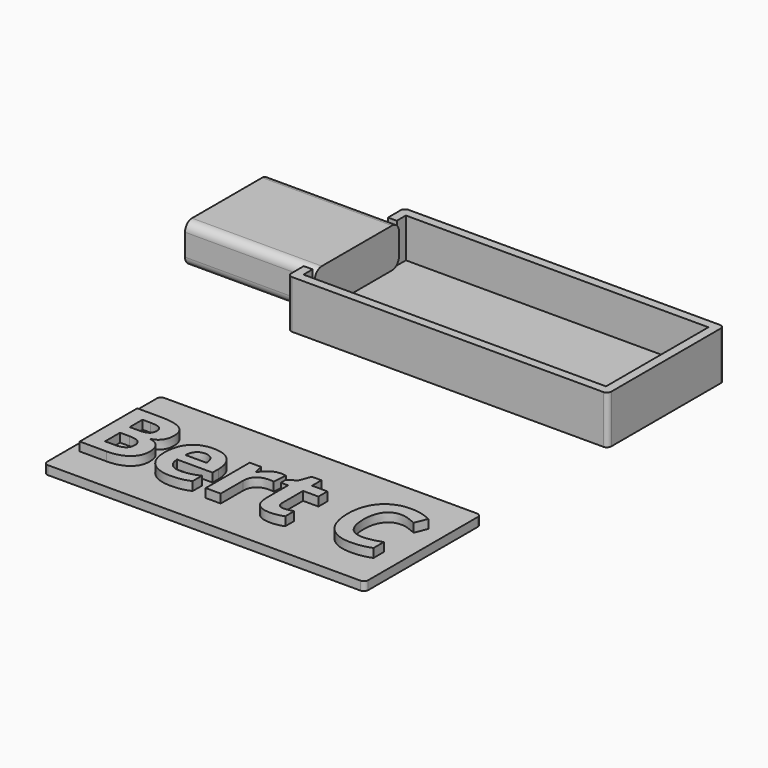
from build123d import *

# Parameters (mm, degrees)
F0_W         = 14.8
F0_H         = 6
F1_DEPTH     = 4.5
F2_R         = 1
F4_W         = 36.5
F4_H         = 16.6
F5_DEPTH     = 1
F6_DEPTH     = 4.5
F7_DEPTH     = 2
F8_R         = 0.5
F9_W         = 36.6
F9_H         = 16.6
F9_TEXT_SIZE = 11.4848814895
F10_DEPTH    = 1
F11_DEPTH    = 1
F12_R        = 0.5


# Not quite as in the source:
# - Text() gives the source's letters only with a copy of the font that has no kerning and outlines rounded to 1/6400 em; it was checked with that copy


with BuildPart() as f1:
    # F0 (on Top) → F1 (new body)
    with BuildSketch(Plane.XY):
        with Locations((-28.2312738687, -1.3390618086)):
            Rectangle(F0_W, F0_H)
        with Locations((-28.2312738687, -7.3390618086)):
            Rectangle(F0_W, F0_H)
    extrude(amount=F1_DEPTH)

    # F2
    f2_edges = [f1.edges().sort_by_distance(p)[0] for p in [
        (-28.231274, 1.660938, 4.5),
        (-28.231274, 1.660938, 0),
        (-28.231274, -10.339062, 4.5),
        (-28.231274, -10.339062, 0),
    ]]
    fillet(f2_edges, radius=F2_R)


with BuildPart() as f5:
    # F4 (on face) → F5 (new body)
    with BuildSketch(Plane.XY):
        with Locations((-3.8312738687, -4.3390618086)):
            Rectangle(F4_W, F4_H)
    extrude(amount=-F5_DEPTH)

    # F3 (on face) → F6 (join)
    with BuildSketch(Plane.XY):
        Polygon((-21.0812738687, 2.9609381914), (12.6687261313, 2.9609381914), (13.4187261313, 2.9609381914), (13.4187261313, -11.6390618086), (12.6687261313, -11.6390618086), (-21.0812738687, -11.6390618086), (-21.0812738687, -10.3390618086), (-22.0812738687, -10.3390618086), (-22.0812738687, -12.6390618086), (14.4187261313, -12.6390618086), (14.4187261313, 3.9609381914), (-22.0812738687, 3.9609381914), (-22.0812738687, 1.6609381914), (-21.0812738687, 1.6609381914), align=None)
    extrude(amount=F6_DEPTH)

    # F3 (on face) → F7 (join)
    with BuildSketch(Plane.XY):
        Polygon((13.1687261313, 2.7109381914), (12.6687261313, 2.7109381914), (12.6687261313, 2.2109381914), (12.6687261313, -10.8890618086), (12.6687261313, -11.3890618086), (13.1687261313, -11.3890618086), align=None)
        Polygon((12.6687261313, 2.9609381914), (12.6687261313, 2.7109381914), (13.1687261313, 2.7109381914), (13.1687261313, -11.3890618086), (12.6687261313, -11.3890618086), (12.6687261313, -11.6390618086), (13.4187261313, -11.6390618086), (13.4187261313, 2.9609381914), align=None)
    extrude(amount=F7_DEPTH)

    # F8
    f8_edges = [f5.edges().sort_by_distance(p)[0] for p in [
        (-22.081274, -12.639062, 1.75),
        (-22.081274, 3.960938, 1.75),
        (14.418726, 3.960938, 1.75),
        (14.418726, -12.639062, 1.75),
    ]]
    fillet(f8_edges, radius=F8_R)


with BuildPart() as f10:
    # F9 (on face) → F10 (new body)
    with BuildSketch(Plane.XY):
        with Locations((-3.4642541975, -39.5011965752)):
            Rectangle(F9_W, F9_H)
        with BuildLine():
            Line((-20.7324093762, -43.9682173411), (-20.7324093762, -35.7690886653))
            Line((-20.7324093762, -35.7690886653), (-18.1806122702, -35.7690886653))
            add(Edge.make_bspline(
                [(-18.1806122702, -35.7690886653), (-16.436345894, -35.7690886653), (-15.6485548043, -36.2652714359)],
                knots=[0, 0, 0, 1, 1, 1], degree=2))
            add(Edge.make_bspline(
                [(-15.6485548043, -36.2652714359), (-14.8607637146, -36.7614542065), (-14.8607637146, -37.8435453843)],
                knots=[0, 0, 0, 1, 1, 1], degree=2))
            add(Edge.make_bspline(
                [(-14.8607637146, -37.8435453843), (-14.8607637146, -38.5792956047), (-15.2053101593, -39.0503551971)],
                knots=[0, 0, 0, 1, 1, 1], degree=2))
            add(Edge.make_bspline(
                [(-15.2053101593, -39.0503551971), (-15.549856604, -39.5214147894), (-16.1223061657, -39.6165239642)],
                knots=[0, 0, 0, 1, 1, 1], degree=2))
            Line((-16.1223061657, -39.6165239642), (-16.1223061657, -39.672153859))
            add(Edge.make_bspline(
                [(-16.1223061657, -39.672153859), (-15.3434876397, -39.846221594), (-14.9980439387, -40.3226647246)],
                knots=[0, 0, 0, 1, 1, 1], degree=2))
            add(Edge.make_bspline(
                [(-14.9980439387, -40.3226647246), (-14.6526002376, -40.7991078551), (-14.6526002376, -41.5904879703)],
                knots=[0, 0, 0, 1, 1, 1], degree=2))
            add(Edge.make_bspline(
                [(-14.6526002376, -41.5904879703), (-14.6526002376, -42.7120584282), (-15.4637199928, -43.3401378847)],
                knots=[0, 0, 0, 1, 1, 1], degree=2))
            add(Edge.make_bspline(
                [(-15.4637199928, -43.3401378847), (-16.274839748, -43.9682173411), (-17.6655871159, -43.9682173411)],
                knots=[0, 0, 0, 1, 1, 1], degree=2))
            Line((-17.6655871159, -43.9682173411), (-20.7324093762, -43.9682173411))
        make_face(mode=Mode.SUBTRACT)
        with BuildLine():
            add(Edge.make_bspline(
                [(-9.0680766133, -43.9718063666), (-9.5777182294, -44.0812716433), (-10.3134684499, -44.0812716433)],
                knots=[0, 0, 0, 1, 1, 1], degree=2))
            add(Edge.make_bspline(
                [(-10.3134684499, -44.0812716433), (-11.8262426836, -44.0812716433), (-12.6786362316, -43.2450287099)],
                knots=[0, 0, 0, 1, 1, 1], degree=2))
            add(Edge.make_bspline(
                [(-12.6786362316, -43.2450287099), (-13.5310297797, -42.4087857764), (-13.5310297797, -40.8780664154)],
                knots=[0, 0, 0, 1, 1, 1], degree=2))
            add(Edge.make_bspline(
                [(-13.5310297797, -40.8780664154), (-13.5310297797, -39.302484236), (-12.74323869, -38.4420153807)],
                knots=[0, 0, 0, 1, 1, 1], degree=2))
            add(Edge.make_bspline(
                [(-12.74323869, -38.4420153807), (-11.9554476003, -37.5815465253), (-10.5647002324, -37.5815465253)],
                knots=[0, 0, 0, 1, 1, 1], degree=2))
            add(Edge.make_bspline(
                [(-10.5647002324, -37.5815465253), (-9.2367608102, -37.5815465253), (-8.4965243079, -38.3379336422)],
                knots=[0, 0, 0, 1, 1, 1], degree=2))
            add(Edge.make_bspline(
                [(-8.4965243079, -38.3379336422), (-7.7562878057, -39.094320759), (-7.7562878057, -40.4294382322)],
                knots=[0, 0, 0, 1, 1, 1], degree=2))
            Line((-7.7562878057, -40.4294382322), (-7.7562878057, -41.2602976274))
            Line((-7.7562878057, -41.2602976274), (-11.7993249926, -41.2602976274))
            add(Edge.make_bspline(
                [(-11.7993249926, -41.2602976274), (-11.7706127888, -41.9888697969), (-11.366847424, -42.3980187)],
                knots=[0, 0, 0, 1, 1, 1], degree=2))
            add(Edge.make_bspline(
                [(-11.366847424, -42.3980187), (-10.9630820591, -42.8071676031), (-10.2345098896, -42.8071676031)],
                knots=[0, 0, 0, 1, 1, 1], degree=2))
            add(Edge.make_bspline(
                [(-10.2345098896, -42.8071676031), (-9.6674438661, -42.8071676031), (-9.1631857882, -42.6896270191)],
                knots=[0, 0, 0, 1, 1, 1], degree=2))
            add(Edge.make_bspline(
                [(-9.1631857882, -42.6896270191), (-8.6589277103, -42.5720864351), (-8.109806814, -42.3136766016)],
                knots=[0, 0, 0, 1, 1, 1], degree=2))
            Line((-8.109806814, -42.3136766016), (-8.109806814, -43.6380269983))
            add(Edge.make_bspline(
                [(-8.109806814, -43.6380269983), (-8.5584349972, -43.8623410899), (-9.0680766133, -43.9718063666)],
                knots=[0, 0, 0, 1, 1, 1], degree=2))
        make_face(mode=Mode.SUBTRACT)
        with BuildLine():
            add(Edge.make_bspline(
                [(-3.9456400177, -37.9036615608), (-3.4494572471, -37.5815465253), (-2.866240609, -37.5815465253)],
                knots=[0, 0, 0, 1, 1, 1], degree=2))
            add(Edge.make_bspline(
                [(-2.866240609, -37.5815465253), (-2.5181051388, -37.5815465253), (-2.288407509, -37.6317928818)],
                knots=[0, 0, 0, 1, 1, 1], degree=2))
            Line((-2.288407509, -37.6317928818), (-2.4176124258, -39.2342927522))
            add(Edge.make_bspline(
                [(-2.4176124258, -39.2342927522), (-2.6257759028, -39.1786628575), (-2.9218705037, -39.1786628575)],
                knots=[0, 0, 0, 1, 1, 1], degree=2))
            add(Edge.make_bspline(
                [(-2.9218705037, -39.1786628575), (-3.7401683098, -39.1786628575), (-4.1977690567, -39.5994760933)],
                knots=[0, 0, 0, 1, 1, 1], degree=2))
            add(Edge.make_bspline(
                [(-4.1977690567, -39.5994760933), (-4.6553698035, -40.0202893291), (-4.6553698035, -40.7775737023)],
                knots=[0, 0, 0, 1, 1, 1], degree=2))
            Line((-4.6553698035, -40.7775737023), (-4.6553698035, -43.9682173411))
            Line((-4.6553698035, -43.9682173411), (-6.3655404378, -43.9682173411))
            Line((-6.3655404378, -43.9682173411), (-6.3655404378, -37.6981898529))
            Line((-6.3655404378, -37.6981898529), (-5.0699022448, -37.6981898529))
            Line((-5.0699022448, -37.6981898529), (-4.8168759495, -38.7533633398))
            Line((-4.8168759495, -38.7533633398), (-4.7343283638, -38.7533633398))
            add(Edge.make_bspline(
                [(-4.7343283638, -38.7533633398), (-4.4418227883, -38.2257765964), (-3.9456400177, -37.9036615608)],
                knots=[0, 0, 0, 1, 1, 1], degree=2))
        make_face(mode=Mode.SUBTRACT)
        with BuildLine():
            add(Edge.make_bspline(
                [(0.9488934608, -42.5433742314), (1.1534679124, -42.7174419664), (1.4908363061, -42.7174419664)],
                knots=[0, 0, 0, 1, 1, 1], degree=2))
            add(Edge.make_bspline(
                [(1.4908363061, -42.7174419664), (1.9394644893, -42.7174419664), (2.5675439458, -42.5218400786)],
                knots=[0, 0, 0, 1, 1, 1], degree=2))
            Line((2.5675439458, -42.5218400786), (2.5675439458, -43.7941496061))
            add(Edge.make_bspline(
                [(2.5675439458, -43.7941496061), (1.9286974129, -44.0812716433), (0.9973453046, -44.0812716433)],
                knots=[0, 0, 0, 1, 1, 1], degree=2))
            add(Edge.make_bspline(
                [(0.9973453046, -44.0812716433), (-0.0291159785, -44.0812716433), (-0.4974838018, -43.5617602072)],
                knots=[0, 0, 0, 1, 1, 1], degree=2))
            add(Edge.make_bspline(
                [(-0.4974838018, -43.5617602072), (-0.965851625, -43.0422487711), (-0.965851625, -42.0050204115)],
                knots=[0, 0, 0, 1, 1, 1], degree=2))
            Line((-0.965851625, -42.0050204115), (-0.965851625, -38.9830609696))
            Line((-0.965851625, -38.9830609696), (-1.7841494311, -38.9830609696))
            Line((-1.7841494311, -38.9830609696), (-1.7841494311, -38.2598723383))
            Line((-1.7841494311, -38.2598723383), (-0.8420302464, -37.6874227766))
            Line((-0.8420302464, -37.6874227766), (-0.3485392449, -36.3630723798))
            Line((-0.3485392449, -36.3630723798), (0.7443190093, -36.3630723798))
            Line((0.7443190093, -36.3630723798), (0.7443190093, -37.6981898529))
            Line((0.7443190093, -37.6981898529), (2.4993524619, -37.6981898529))
            Line((2.4993524619, -37.6981898529), (2.4993524619, -38.9830609696))
            Line((2.4993524619, -38.9830609696), (0.7443190093, -38.9830609696))
            Line((0.7443190093, -38.9830609696), (0.7443190093, -42.0050204115))
            add(Edge.make_bspline(
                [(0.7443190093, -42.0050204115), (0.7443190093, -42.3693064963), (0.9488934608, -42.5433742314)],
                knots=[0, 0, 0, 1, 1, 1], degree=2))
        make_face(mode=Mode.SUBTRACT)
        with BuildLine():
            add(Edge.make_bspline(
                [(11.3498892598, -37.2612260025), (10.885110462, -37.0988226002), (10.4364822788, -37.0988226002)],
                knots=[0, 0, 0, 1, 1, 1], degree=2))
            add(Edge.make_bspline(
                [(10.4364822788, -37.0988226002), (9.454883814, -37.0988226002), (8.9165299942, -37.8363673334)],
                knots=[0, 0, 0, 1, 1, 1], degree=2))
            add(Edge.make_bspline(
                [(8.9165299942, -37.8363673334), (8.3781761744, -38.5739120665), (8.3781761744, -39.8910844124)],
                knots=[0, 0, 0, 1, 1, 1], degree=2))
            add(Edge.make_bspline(
                [(8.3781761744, -39.8910844124), (8.3781761744, -42.633099868), (10.4364822788, -42.633099868)],
                knots=[0, 0, 0, 1, 1, 1], degree=2))
            add(Edge.make_bspline(
                [(10.4364822788, -42.633099868), (11.2996429033, -42.633099868), (12.5270896125, -42.2024168121)],
                knots=[0, 0, 0, 1, 1, 1], degree=2))
            Line((12.5270896125, -42.2024168121), (12.5270896125, -43.6595611511))
            add(Edge.make_bspline(
                [(12.5270896125, -43.6595611511), (11.5185734567, -44.0812716433), (10.2731816202, -44.0812716433)],
                knots=[0, 0, 0, 1, 1, 1], degree=2))
            add(Edge.make_bspline(
                [(10.2731816202, -44.0812716433), (8.4840524256, -44.0812716433), (7.5365497027, -42.99559144)],
                knots=[0, 0, 0, 1, 1, 1], degree=2))
            add(Edge.make_bspline(
                [(7.5365497027, -42.99559144), (6.5890469798, -41.9099112367), (6.5890469798, -39.880317336)],
                knots=[0, 0, 0, 1, 1, 1], degree=2))
            add(Edge.make_bspline(
                [(6.5890469798, -39.880317336), (6.5890469798, -38.6008297575), (7.054723034, -37.6389709328)],
                knots=[0, 0, 0, 1, 1, 1], degree=2))
            add(Edge.make_bspline(
                [(7.054723034, -37.6389709328), (7.5203990881, -36.677112108), (8.3925322763, -36.1647787228)],
                knots=[0, 0, 0, 1, 1, 1], degree=2))
            add(Edge.make_bspline(
                [(8.3925322763, -36.1647787228), (9.2646654644, -35.6524453376), (10.4364822788, -35.6524453376)],
                knots=[0, 0, 0, 1, 1, 1], degree=2))
            add(Edge.make_bspline(
                [(10.4364822788, -35.6524453376), (11.6298332461, -35.6524453376), (12.8357458025, -36.2284839248)],
                knots=[0, 0, 0, 1, 1, 1], degree=2))
            Line((12.8357458025, -36.2284839248), (12.2758578299, -37.6425599582))
            add(Edge.make_bspline(
                [(12.2758578299, -37.6425599582), (11.8146680576, -37.4236294048), (11.3498892598, -37.2612260025)],
                knots=[0, 0, 0, 1, 1, 1], degree=2))
        make_face(mode=Mode.SUBTRACT)
        with Locations((-21.7642541975, -43.9682173411)):
            Text('Bert C', F9_TEXT_SIZE, font='Open Sans', font_style=FontStyle.BOLD, text_align=(TextAlign.LEFT, TextAlign.BOTTOM))
        with BuildLine():
            Line((-17.9168188985, -40.3953424903), (-18.9935265381, -40.3953424903))
            Line((-18.9935265381, -40.3953424903), (-18.9935265381, -42.532607155))
            Line((-18.9935265381, -42.532607155), (-17.8611890038, -42.532607155))
            add(Edge.make_bspline(
                [(-17.8611890038, -42.532607155), (-17.1433839107, -42.532607155), (-16.8015292351, -42.2580467068)],
                knots=[0, 0, 0, 1, 1, 1], degree=2))
            add(Edge.make_bspline(
                [(-16.8015292351, -42.2580467068), (-16.4596745595, -41.9834862587), (-16.4596745595, -41.4164202352)],
                knots=[0, 0, 0, 1, 1, 1], degree=2))
            add(Edge.make_bspline(
                [(-16.4596745595, -41.4164202352), (-16.4596745595, -40.3953424903), (-17.9168188985, -40.3953424903)],
                knots=[0, 0, 0, 1, 1, 1], degree=2))
        make_face()
        with BuildLine():
            Line((-18.9935265381, -37.193931775), (-18.9935265381, -39.0171567115))
            Line((-18.9935265381, -39.0171567115), (-17.9850103823, -39.0171567115))
            add(Edge.make_bspline(
                [(-17.9850103823, -39.0171567115), (-17.2779723656, -39.0171567115), (-16.9612408683, -38.7982261581)],
                knots=[0, 0, 0, 1, 1, 1], degree=2))
            add(Edge.make_bspline(
                [(-16.9612408683, -38.7982261581), (-16.644509371, -38.5792956047), (-16.644509371, -38.0750375268)],
                knots=[0, 0, 0, 1, 1, 1], degree=2))
            add(Edge.make_bspline(
                [(-16.644509371, -38.0750375268), (-16.644509371, -37.6030806781), (-16.9890558157, -37.3985062266)],
                knots=[0, 0, 0, 1, 1, 1], degree=2))
            add(Edge.make_bspline(
                [(-16.9890558157, -37.3985062266), (-17.3336022603, -37.193931775), (-18.0801195572, -37.193931775)],
                knots=[0, 0, 0, 1, 1, 1], degree=2))
            Line((-18.0801195572, -37.193931775), (-18.9935265381, -37.193931775))
        make_face()
        with BuildLine():
            add(Edge.make_bspline(
                [(-9.6907725316, -39.1427726028), (-10.010195798, -38.7982261581), (-10.553933156, -38.7982261581)],
                knots=[0, 0, 0, 1, 1, 1], degree=2))
            add(Edge.make_bspline(
                [(-10.553933156, -38.7982261581), (-11.0976705141, -38.7982261581), (-11.4063267041, -39.1427726028)],
                knots=[0, 0, 0, 1, 1, 1], degree=2))
            add(Edge.make_bspline(
                [(-11.4063267041, -39.1427726028), (-11.7149828941, -39.4873190475), (-11.7598457124, -40.1207820422)],
                knots=[0, 0, 0, 1, 1, 1], degree=2))
            Line((-11.7598457124, -40.1207820422), (-9.358787676, -40.1207820422))
            add(Edge.make_bspline(
                [(-9.358787676, -40.1207820422), (-9.3713492652, -39.4873190475), (-9.6907725316, -39.1427726028)],
                knots=[0, 0, 0, 1, 1, 1], degree=2))
        make_face()
    extrude(amount=-F10_DEPTH)

    # F9 (on face) → F11 (join)
    with BuildSketch(Plane.XY):
        with Locations((-21.7642541975, -43.9682173411)):
            Text('Bert C', F9_TEXT_SIZE, font='Open Sans', font_style=FontStyle.BOLD, text_align=(TextAlign.LEFT, TextAlign.BOTTOM))
    extrude(amount=F11_DEPTH)

    # F12
    f12_edges = [f10.edges().sort_by_distance(p)[0] for p in [
        (-21.764254, -47.801197, -0.5),
        (14.835746, -47.801197, -0.5),
        (14.835746, -31.201197, -0.5),
        (-21.764254, -31.201197, -0.5),
    ]]
    fillet(f12_edges, radius=F12_R)


solid = Compound([f1.part, f5.part, f10.part])
